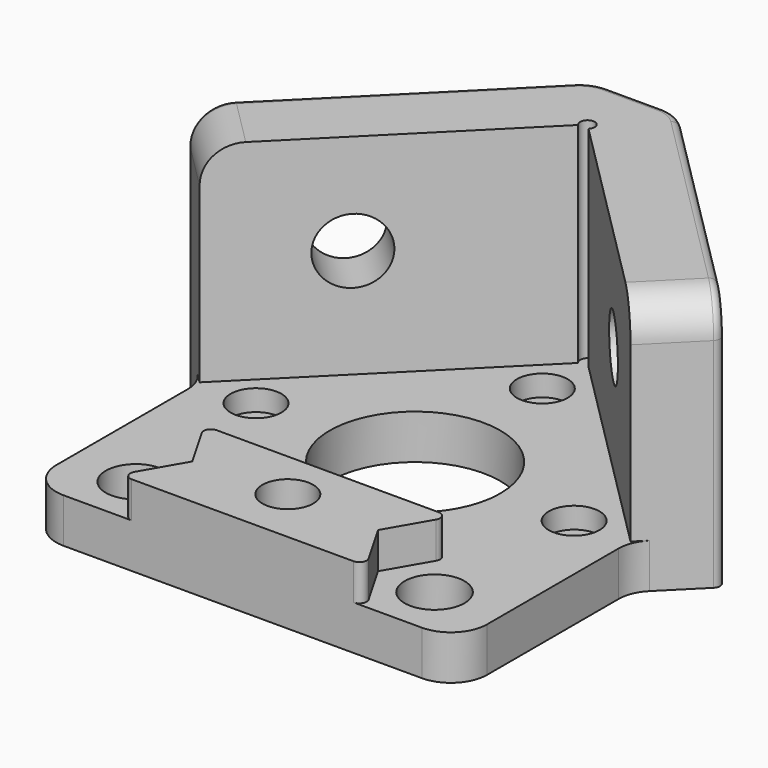
from build123d import *

# Parameters (mm, degrees)
F0_R          = 4.125
F0_R_2        = 1.7
F0_R_3        = 11.75
F1_DEPTH      = 6.13
F3_DEPTH      = 35
F4_R          = 4.5
F5_DEPTH      = 10
F6_R          = 4.25
F7_DEPTH      = 10
F8_R          = 7
F9_DEPTH      = 3
F10_R         = 7
F11_DEPTH     = 3
F13_R         = 5
F12_R         = 3.5
F14_DEPTH     = 2.9
F15_R         = 3.5
F16_DEPTH     = 5
F17_T1_DEPTH  = 32.5
F17_T3_DEPTH  = 9.3301270189
F17_T5_DEPTH  = 36.6690475583
F17_T7_DEPTH  = 7.5391052434
F17_T9_DEPTH  = 36.6690475583
F17_T12_ANGLE = 90
F17_T14_ANGLE = 45
F17_T16_ANGLE = 45
F17_T18_ANGLE = 90
F18_R         = 1
F19_DEPTH     = 28.87


# Not quite as in the source:
# - a fillet or chamfer that OpenCascade refuses, or shapes differently, is made with other operations: its cross-section is extruded or revolved along the edge and cut away or added


with BuildPart() as f1:
    # F0 (on Top) → F1 (new body)
    with BuildSketch(Plane.XY):
        Polygon((-29.6984848098, 0), (0, 0), (29.6984848098, 0), (29.6984848098, 29.7), (0, 59.3984848098), (-29.6984848098, 29.7), align=None)
        with Locations((-20.59, 7.3196897832)):
            Circle(F0_R, mode=Mode.SUBTRACT)
        with Locations((0, 7.7796897832)):
            Circle(F0_R_2, mode=Mode.SUBTRACT)
        with Locations((20.59, 7.3196897832)):
            Circle(F0_R, mode=Mode.SUBTRACT)
        with Locations((-21.9203102168, 29.7)):
            Circle(F0_R_2, mode=Mode.SUBTRACT)
        with Locations((0, 29.7)):
            Circle(F0_R_3, mode=Mode.SUBTRACT)
        with Locations((21.9203102168, 29.7)):
            Circle(F0_R_2, mode=Mode.SUBTRACT)
        with Locations((0, 51.6203102168)):
            Circle(F0_R_2, mode=Mode.SUBTRACT)
    extrude(amount=F1_DEPTH)

    # F2 (on face) → F3 (join)
    with BuildSketch(Plane(origin=(0, 0, 0), x_dir=(1, 0, 0), z_dir=(0, 0, -1))):
        Polygon((0, -59.3984848098), (-29.6984848098, -29.7), (-36.7695526217, -36.7710678119), (-5.8406204336, -67.7), (0, -67.7), (5.8406204336, -67.7), (36.7695526217, -36.7710678119), (29.6984848098, -29.7), align=None)
    extrude(amount=-F3_DEPTH)

    # F4 (on face) → F5 (cut, through all)
    with BuildSketch(Plane(origin=(-29.6992424049, 29.6992424049, 0), x_dir=(0.7071067812, 0.7071067812, 0), z_dir=(0.7071067812, -0.7071067812, 0))):
        with Locations((16.6010714012, 21.13)):
            Circle(F4_R)
    extrude(amount=-F5_DEPTH, mode=Mode.SUBTRACT)

    # F6 (on face) → F7 (cut, through all)
    with BuildSketch(Plane(origin=(29.6992424049, 29.6992424049, 0), x_dir=(0.7071067812, -0.7071067812, 0), z_dir=(-0.7071067812, -0.7071067812, 0))):
        with Locations((-16.6010714012, 21.13)):
            Circle(F6_R)
    extrude(amount=-F7_DEPTH, mode=Mode.SUBTRACT)

    # F8 (on face) → F9 (cut)
    with BuildSketch(Plane(origin=(-36.7703102168, 36.7703102168, 0), x_dir=(-0.7071067812, -0.7071067812, 0), z_dir=(-0.7071067812, 0.7071067812, 0))):
        with Locations((-16.6010714006, 21.13)):
            Circle(F8_R)
    extrude(amount=-F9_DEPTH, mode=Mode.SUBTRACT)

    # F10 (on face) → F11 (cut)
    with BuildSketch(Plane(origin=(36.7703102168, 36.7703102168, 0), x_dir=(-0.7071067812, 0.7071067812, 0), z_dir=(0.7071067812, 0.7071067812, 0))):
        with Locations((16.6010714007, 21.13)):
            Circle(F10_R)
    extrude(amount=-F11_DEPTH, mode=Mode.SUBTRACT)

    # F13
    f13_edges = [f1.edges().sort_by_distance(p)[0] for p in [
        (33.234019, 33.235534, 35),
        (-33.234019, 33.235534, 35),
        (29.698485, 29.7, 3.065),
        (29.698485, 0, 3.065),
        (-29.698485, 0, 3.065),
        (-29.698485, 29.7, 3.065),
        (-5.84062, 67.7, 17.5),
        (5.84062, 67.7, 17.5),
    ]]
    fillet(f13_edges, radius=F13_R)

    # F12 (on face) → F14 (cut)
    with BuildSketch(Plane.XY.offset(6.13)):
        with Locations((0, 51.6203102168)):
            Circle(F12_R)
        with Locations((-21.9203102168, 29.7)):
            Circle(F12_R)
        with Locations((21.9203102168, 29.7)):
            Circle(F12_R)
        with Locations((0, 7.7796897832)):
            Circle(F12_R)
    extrude(amount=-F14_DEPTH, mode=Mode.SUBTRACT)

    # F15 (on face) → F16 (join)
    with BuildSketch(Plane.XY.offset(6.13)):
        Polygon((16.692885683, 14.0696897832), (-16.692885683, 14.0696897832), (-12.7957713659, 7.3196897832), (-16.692885683, 0.5696897832), (16.692885683, 0.5696897832), (12.7957713659, 7.3196897832), align=None)
        with Locations((0, 7.7796897832)):
            Circle(F15_R, mode=Mode.SUBTRACT)
        Polygon((16.692885683, 0.5696897832), (-16.692885683, 0.5696897832), (-17.0217962327, 0), (0, 0), (17.0217962327, 0), align=None)
        Polygon((-17.0217962327, 14.6393795664), (-16.692885683, 14.0696897832), (16.692885683, 14.0696897832), (17.0217962327, 14.6393795664), (0, 14.6393795664), align=None)
    extrude(amount=F16_DEPTH)

    # F17: fillet of radius 1 on 13 edges, made by hand

    # F17_s2 → F17_t1 (cut)
    with BuildSketch(Plane.XY.offset(-2.5)):
        with BuildLine():
            ThreePointArc((36.0624458405, 37.4781745931), (36.3553390593, 36.7710678119), (36.0624458405, 36.0639610307))
            Line((36.0624458405, 36.0639610307), (36.7695526217, 36.7710678119))
            Line((36.7695526217, 36.7710678119), (36.0624458405, 37.4781745931))
        make_face()
        with BuildLine():
            ThreePointArc((-36.0624458405, 36.0639610307), (-36.3553390593, 36.7710678119), (-36.0624458405, 37.4781745931))
            Line((-36.0624458405, 37.4781745931), (-36.7695526217, 36.7710678119))
            Line((-36.7695526217, 36.7710678119), (-36.0624458405, 36.0639610307))
        make_face()
    extrude(amount=F17_T1_DEPTH, mode=Mode.SUBTRACT)

    # F17_s4 → F17_t3 (cut)
    with BuildSketch(Plane.XY.offset(6.13)):
        with BuildLine():
            ThreePointArc((-15.2897454251, 0), (-16.1557708289, 0.5), (-16.1557708289, 1.5))
            Line((-16.1557708289, 1.5), (-17.0217962327, 0))
            Line((-17.0217962327, 0), (-15.2897454251, 0))
        make_face()
        with BuildLine():
            ThreePointArc((-15.2897454251, 14.6393795664), (-16.1557708289, 14.1393795664), (-16.1557708289, 13.1393795664))
            Line((-16.1557708289, 13.1393795664), (-17.0217962327, 14.6393795664))
            Line((-17.0217962327, 14.6393795664), (-15.2897454251, 14.6393795664))
        make_face()
        with BuildLine():
            ThreePointArc((16.1557708289, 13.1393795664), (16.1557708289, 14.1393795664), (15.2897454251, 14.6393795664))
            Line((15.2897454251, 14.6393795664), (17.0217962327, 14.6393795664))
            Line((17.0217962327, 14.6393795664), (16.1557708289, 13.1393795664))
        make_face()
        with BuildLine():
            ThreePointArc((15.2897454251, 0), (16.1557708289, 0.5), (16.1557708289, 1.5))
            Line((16.1557708289, 1.5), (17.0217962327, 0))
            Line((17.0217962327, 0), (15.2897454251, 0))
        make_face()
    extrude(amount=F17_T3_DEPTH, mode=Mode.SUBTRACT)

    # F17_s6 → F17_t5 (cut)
    with BuildSketch(Plane(origin=(3.536291501, 3.536291501, 0), x_dir=(0, 0, 1), z_dir=(0.7071067812, 0.7071067812, 0))):
        with BuildLine():
            ThreePointArc((34, -52.0010714012), (34.7071067812, -51.7081781824), (35, -51.0010714012))
            Line((35, -51.0010714012), (35, -52.0010714012))
            Line((35, -52.0010714012), (34, -52.0010714012))
        make_face()
    extrude(amount=F17_T5_DEPTH, mode=Mode.SUBTRACT)

    # F17_s8 → F17_t7 (cut)
    with BuildSketch(Plane.YZ.offset(-3.7695526217)):
        with BuildLine():
            ThreePointArc((67.7, 34), (67.4071067812, 34.7071067812), (66.7, 35))
            Line((66.7, 35), (67.7, 35))
            Line((67.7, 35), (67.7, 34))
        make_face()
    extrude(amount=F17_T7_DEPTH, mode=Mode.SUBTRACT)

    # F17_s10 → F17_t9 (cut)
    with BuildSketch(Plane(origin=(-29.4652236891, 29.4652236891, 0), x_dir=(0, 0, 1), z_dir=(0.7071067812, -0.7071067812, 0))):
        with BuildLine():
            ThreePointArc((34, -52.0010714012), (34.7071067812, -51.7081781824), (35, -51.0010714012))
            Line((35, -51.0010714012), (35, -52.0010714012))
            Line((35, -52.0010714012), (34, -52.0010714012))
        make_face()
    extrude(amount=F17_T9_DEPTH, mode=Mode.SUBTRACT)

    # F17_s11 → F17_t12 (revolve, cut)
    with BuildSketch(Plane.XY.offset(30)):
        with BuildLine():
            ThreePointArc((-36.0624458405, 37.4781745931), (-36.3553390593, 36.7710678119), (-36.0624458405, 36.0639610307))
            Line((-36.0624458405, 36.0639610307), (-36.7695526217, 36.7710678119))
            Line((-36.7695526217, 36.7710678119), (-36.0624458405, 37.4781745931))
        make_face()
    revolve(axis=Axis((-33.2340187158, 40.3066017178, 30), (-0.7071067812, 0.7071067812, 0)), revolution_arc=F17_T12_ANGLE, mode=Mode.SUBTRACT)

    # F17_s13 → F17_t14 (revolve, cut)
    with BuildSketch(Plane.YZ.offset(-3.7695526217)):
        with BuildLine():
            ThreePointArc((67.7, 34), (67.4071067812, 34.7071067812), (66.7, 35))
            Line((66.7, 35), (67.7, 35))
            Line((67.7, 35), (67.7, 34))
        make_face()
    revolve(axis=Axis((-3.7695526217, 62.7, 35), (0, 0, 1)), revolution_arc=F17_T14_ANGLE, mode=Mode.SUBTRACT)

    # F17_s15 → F17_t16 (revolve, cut)
    with BuildSketch(Plane(origin=(-29.4652236891, 29.4652236891, 0), x_dir=(0, 0, 1), z_dir=(0.7071067812, -0.7071067812, 0))):
        with BuildLine():
            ThreePointArc((34, -52.0010714012), (34.7071067812, -51.7081781824), (35, -51.0010714012))
            Line((35, -51.0010714012), (35, -52.0010714012))
            Line((35, -52.0010714012), (34, -52.0010714012))
        make_face()
    revolve(axis=Axis((3.7695526217, 62.7, 35), (0, 0, 1)), revolution_arc=F17_T16_ANGLE, mode=Mode.SUBTRACT)

    # F17_s17 → F17_t18 (revolve, cut)
    with BuildSketch(Plane.XY.offset(30)):
        with BuildLine():
            ThreePointArc((36.0624458405, 37.4781745931), (36.3553390593, 36.7710678119), (36.0624458405, 36.0639610307))
            Line((36.0624458405, 36.0639610307), (36.7695526217, 36.7710678119))
            Line((36.7695526217, 36.7710678119), (36.0624458405, 37.4781745931))
        make_face()
    revolve(axis=Axis((33.2340187158, 40.3066017178, 30), (-0.7071067812, -0.7071067812, 0)), revolution_arc=F17_T18_ANGLE, mode=Mode.SUBTRACT)

    # F18 (on face) → F19 (cut, through all)
    with BuildSketch(Plane.XY.offset(35)):
        with Locations((0, 59.3984848098)):
            Circle(F18_R)
    extrude(amount=-F19_DEPTH, mode=Mode.SUBTRACT)


solid = f1.part
